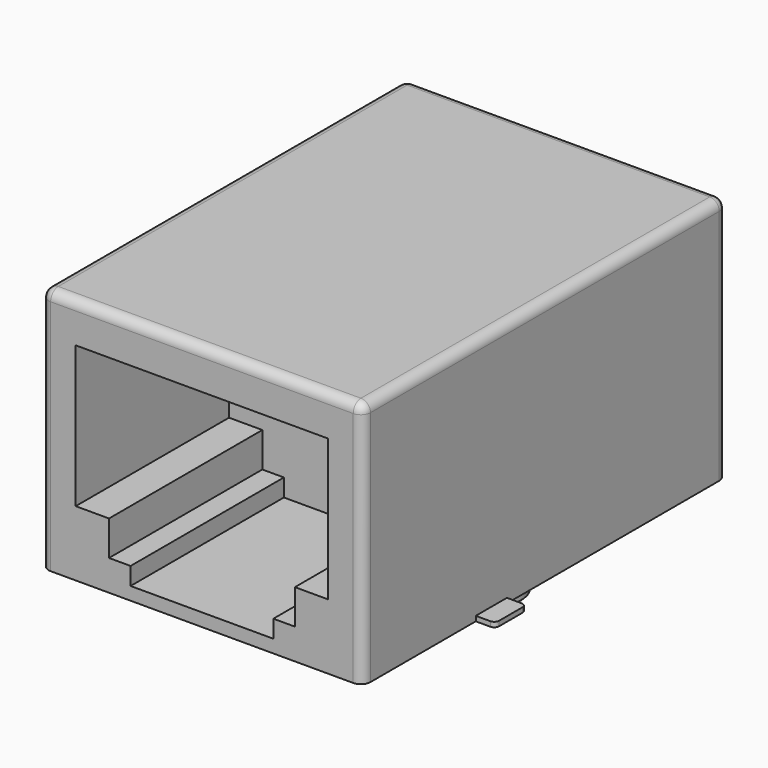
from build123d import *

# Parameters (mm, degrees)
F0_W     = 16.7894
F0_H     = 23.749
F1_DEPTH = 12.8778
F2_R     = 0.5
F4_DEPTH = 10
F5_R     = 1.5875
F6_DEPTH = 0.9906
F7_W     = 0.6096
F7_H     = 1.397
F8_DEPTH = 0.254
F9_SIZE  = 0.381


with BuildPart() as f1:
    # F0 (on Top) → F1 (new body)
    with BuildSketch(Plane.XY):
        Rectangle(F0_W, F0_H)
    extrude(amount=F1_DEPTH)

    # F2
    f2_edges = [f1.edges().sort_by_distance(p)[0] for p in [
        (8.3947, 11.8745, 6.4389),
        (-8.3947, 11.8745, 6.4389),
        (0, -11.8745, 12.8778),
        (-8.3947, 0, 12.8778),
        (0, 11.8745, 12.8778),
        (8.3947, 0, 12.8778),
        (-8.3947, -11.8745, 6.4389),
        (8.3947, -11.8745, 6.4389),
    ]]
    fillet(f2_edges, radius=F2_R)

    # F3 (on face) → F4 (cut)
    with BuildSketch(Plane.XZ.offset(11.8745)):
        Polygon((6.5885786898, 10.8017679304), (0, 10.8017679304), (-6.5885786898, 10.8017679304), (-6.5885786898, 3.4128425177), (-4.8500075936, 3.4128425177), (-4.8500075936, 1.597570139), (-3.7250500172, 1.597570139), (-3.7250500172, 0.6771502085), (0, 0.6771502085), (3.7250500172, 0.6771502085), (3.7250500172, 1.597570139), (4.8500075936, 1.597570139), (4.8500075936, 3.4128425177), (6.5885786898, 3.4128425177), align=None)
    extrude(amount=-F4_DEPTH, mode=Mode.SUBTRACT)

    # F5 (on face) → F6 (join)
    with BuildSketch(Plane(origin=(0, 0, 0), x_dir=(1, 0, 0), z_dir=(0, 0, -1))):
        with Locations((6.35, 0.9525)):
            Circle(F5_R)
        with Locations((-6.35, 0.9525)):
            Circle(F5_R)
    extrude(amount=F6_DEPTH)

    # F7 (on face) → F8 (join)
    with BuildSketch(Plane(origin=(0, 0, 0), x_dir=(1, 0, 0), z_dir=(0, 0, -1))):
        with Locations((1.016, -12.5095)):
            Rectangle(F7_W, F7_H)
        with Locations((3.048, -12.5095)):
            Rectangle(F7_W, F7_H)
        with Locations((5.08, -12.5095)):
            Rectangle(F7_W, F7_H)
        with Locations((-1.016, -12.5095)):
            Rectangle(F7_W, F7_H)
        with Locations((-5.08, -12.5095)):
            Rectangle(F7_W, F7_H)
        with Locations((-3.048, -12.5095)):
            Rectangle(F7_W, F7_H)
        with BuildLine():
            Line((9.1567, 4.5085), (8.3947, 4.5085))
            Line((8.3947, 4.5085), (8.3947, 2.4765))
            Line((8.3947, 2.4765), (9.1567, 2.4765))
            ThreePointArc((9.1567, 2.4765), (9.3363051224, 2.5508948776), (9.4107, 2.7305))
            Line((9.4107, 2.7305), (9.4107, 4.2545))
            ThreePointArc((9.4107, 4.2545), (9.3363051224, 4.4341051224), (9.1567, 4.5085))
        make_face()
        with BuildLine():
            ThreePointArc((-9.1567, 4.5085), (-9.3363051224, 4.4341051224), (-9.4107, 4.2545))
            Line((-9.4107, 4.2545), (-9.4107, 2.7305))
            ThreePointArc((-9.4107, 2.7305), (-9.3363051224, 2.5508948776), (-9.1567, 2.4765))
            Line((-9.1567, 2.4765), (-8.3947, 2.4765))
            Line((-8.3947, 2.4765), (-8.3947, 4.5085))
            Line((-8.3947, 4.5085), (-9.1567, 4.5085))
        make_face()
    extrude(amount=-F8_DEPTH)

    # F9
    f9_edges = [f1.edges().sort_by_distance(p)[0] for p in [
        (4.7625, -0.9525, -0.9906),
        (-7.9375, -0.9525, -0.9906),
    ]]
    chamfer(f9_edges, length=F9_SIZE)


solid = f1.part
